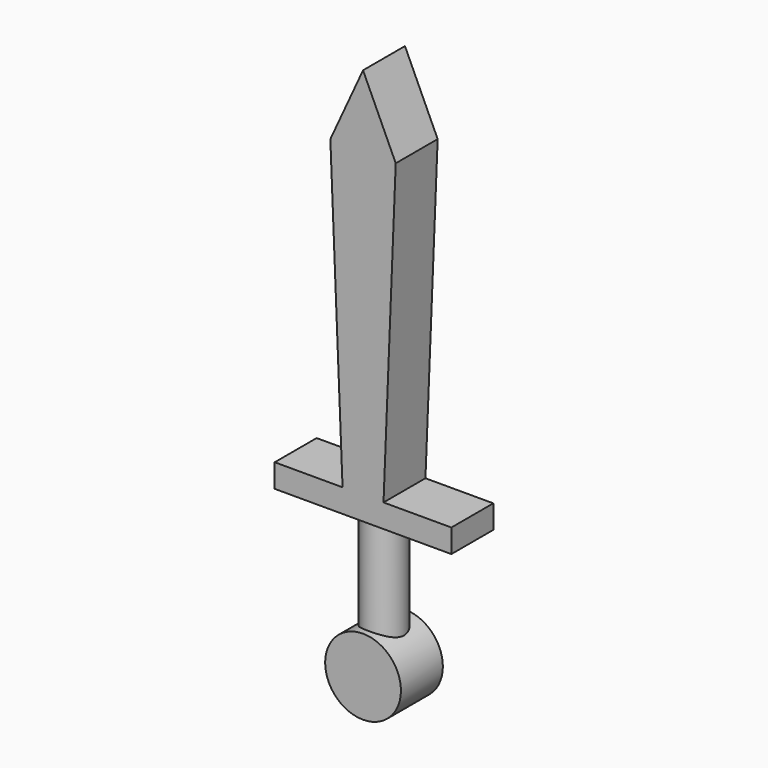
from build123d import *

# Parameters (mm, degrees)
F0_W     = 9.6974931657
F0_H     = 5.6765731424
F0_W_2   = 9.6974670887
F1_DEPTH = 12.7
F3_DEPTH = 12.7


# Not quite as in the source:
# - ends of sketch curves that miss each other by under 0.0002 mm in the source are joined


with BuildPart() as f1:
    # F0 (on Front) → F1 (new body, symmetric)
    with BuildSketch(Plane.XZ):
        Polygon((-9.9266454939, 27.6733003557), (9.9266454939, 27.6733003557), (15.8470887691, 174.3181347847), (0, 208.8506370783), (-15.8470887691, 174.3181347847), align=None)
        Polygon((9.6974931657, 21.9967272133), (9.6974931657, 16.3201540709), (42.8108498454, 16.3201540709), (42.8108498454, 27.6733003557), (9.9266454939, 27.6733003557), align=None)
        Polygon((-42.8108498454, 16.3201540709), (-9.6974670887, 16.3201540709), (-9.6974670887, 21.9967272133), (-9.9266454939, 27.6733003557), (-42.8108498454, 27.6733003557), align=None)
        Polygon((0, 21.9967272133), (9.6974931657, 21.9967272133), (9.9266454939, 27.6733003557), (-9.9266454939, 27.6733003557), (-9.6974670887, 21.9967272133), align=None)
        with Locations((4.8487465829, 19.1584406421)):
            Rectangle(F0_W, F0_H)
        with Locations((-4.8487335443, 19.1584406421)):
            Rectangle(F0_W_2, F0_H)
    extrude(amount=F1_DEPTH, both=True)


with BuildPart() as f2:
    # F0 (on Front) → F2 (revolve)
    with BuildSketch(Plane.XZ):
        with BuildLine():
            ThreePointArc((0, -31.5412492268), (5.0425448571, -32.2470761559), (9.6974931657, -34.3103033691))
            Line((9.6974931657, -34.3103033691), (9.6974931657, 16.3201540709))
            Line((9.6974931657, 16.3201540709), (0, 16.3201540709))
            Line((0, 16.3201540709), (0, -31.5412492268))
        make_face()
    revolve(axis=Axis((0, 0, -14.901005663), (0, 0, 1)))

    # F0 (on Front) → F3 (join, symmetric)
    with BuildSketch(Plane.XZ):
        with BuildLine():
            ThreePointArc((-9.6974670887, -34.3102871549), (-8.9215307642, -65.9592970493), (18.3653026112, -49.9065518379))
            ThreePointArc((18.3653026112, -49.9065518379), (16.0527526698, -40.9850344938), (9.6974931657, -34.3103033691))
            Line((9.6974931657, -34.3103033691), (9.6974931657, -51.7987385392))
            Line((9.6974931657, -51.7987385392), (0, -51.7987385392))
            Line((0, -51.7987385392), (-9.6974670887, -51.7987385392))
            Line((-9.6974670887, -51.7987385392), (-9.6974670887, -34.3102871549))
        make_face()
        with BuildLine():
            ThreePointArc((0, -31.5412492268), (-5.0425300937, -32.2470719403), (-9.6974670887, -34.3102871549))
            Line((-9.6974670887, -34.3102871549), (-9.6974670887, -51.7987385392))
            Line((-9.6974670887, -51.7987385392), (0, -51.7987385392))
            Line((0, -51.7987385392), (0, -49.9065518379))
            Line((0, -49.9065518379), (0, -31.5412492268))
        make_face()
        with BuildLine():
            Line((9.6974931657, -51.7987385392), (9.6974931657, -34.3103033691))
            ThreePointArc((9.6974931657, -34.3103033691), (5.0425448571, -32.2470761559), (0, -31.5412492268))
            Line((0, -31.5412492268), (0, -49.9065518379))
            Line((0, -49.9065518379), (0, -51.7987385392))
            Line((0, -51.7987385392), (9.6974931657, -51.7987385392))
        make_face()
    extrude(amount=F3_DEPTH, both=True)


solid = Compound([f1.part, f2.part])
